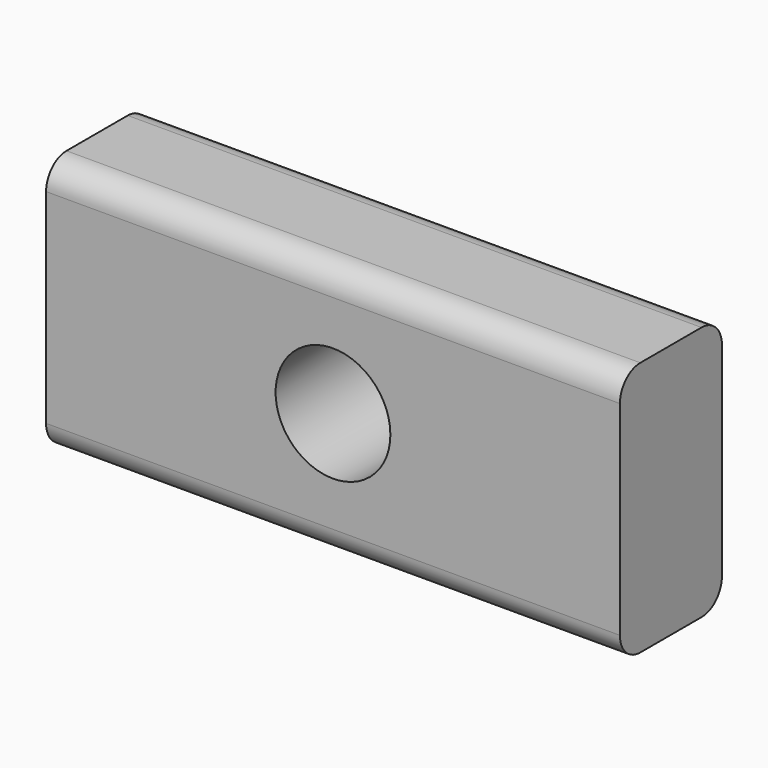
from build123d import *

# Parameters (mm, degrees)
F0_W     = 5
F0_H     = 10
F1_DEPTH = 11.25
F2_R     = 2.25
F3_DEPTH = 5.001
F4_R     = 1


with BuildPart() as f1:
    # F0 (on Right) → F1 (new body, symmetric)
    with BuildSketch(Plane.YZ):
        with Locations((2.5, 0)):
            Rectangle(F0_W, F0_H)
    extrude(amount=F1_DEPTH, both=True)

    # F2 (on face) → F3 (cut, through all)
    with BuildSketch(Plane.XZ):
        Circle(F2_R)
    extrude(amount=-F3_DEPTH, mode=Mode.SUBTRACT)

    # F4
    f4_edges = [f1.edges().sort_by_distance(p)[0] for p in [
        (0, 0, 5),
        (0, 0, -5),
        (0, 5, 5),
        (0, 5, -5),
    ]]
    fillet(f4_edges, radius=F4_R)


solid = f1.part
